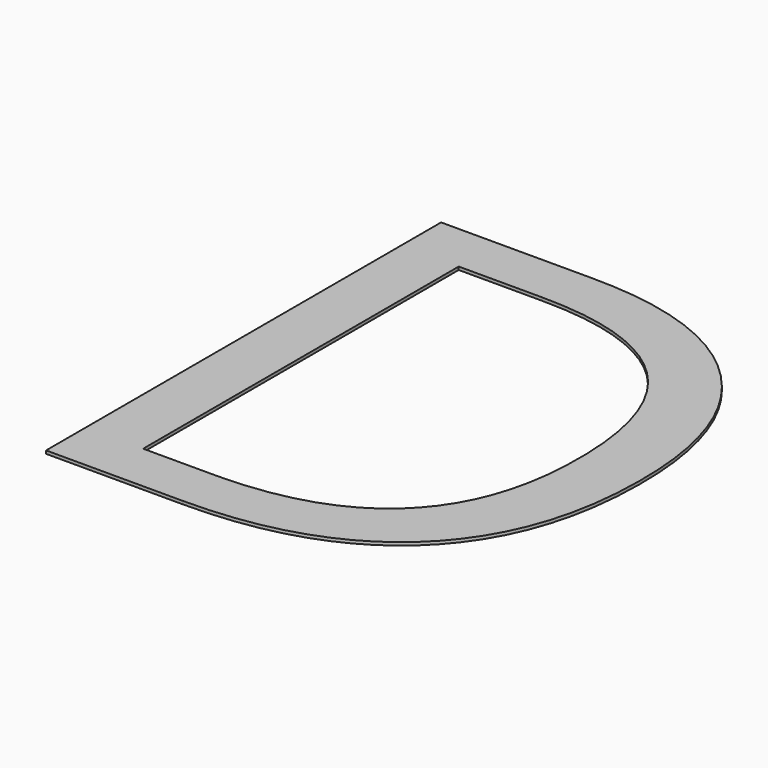
from build123d import *

# Parameters (mm, degrees)
F0_TEXT_SIZE = 45.1796080193
F1_DEPTH     = 0.2


# Not quite as in the source:
# - Text() gives the source's letters only with a copy of the font that has no kerning and outlines rounded to 1/6400 em; it was checked with that copy


with BuildPart() as f1:
    # F0 (on Top) → F1 (new body)
    with BuildSketch(Plane.XY):
        with Locations((-16.5540907508, -32.5293177739)):
            Text('D', F0_TEXT_SIZE, font='Open Sans', text_align=(TextAlign.LEFT, TextAlign.BOTTOM))
    extrude(amount=F1_DEPTH)


solid = f1.part
